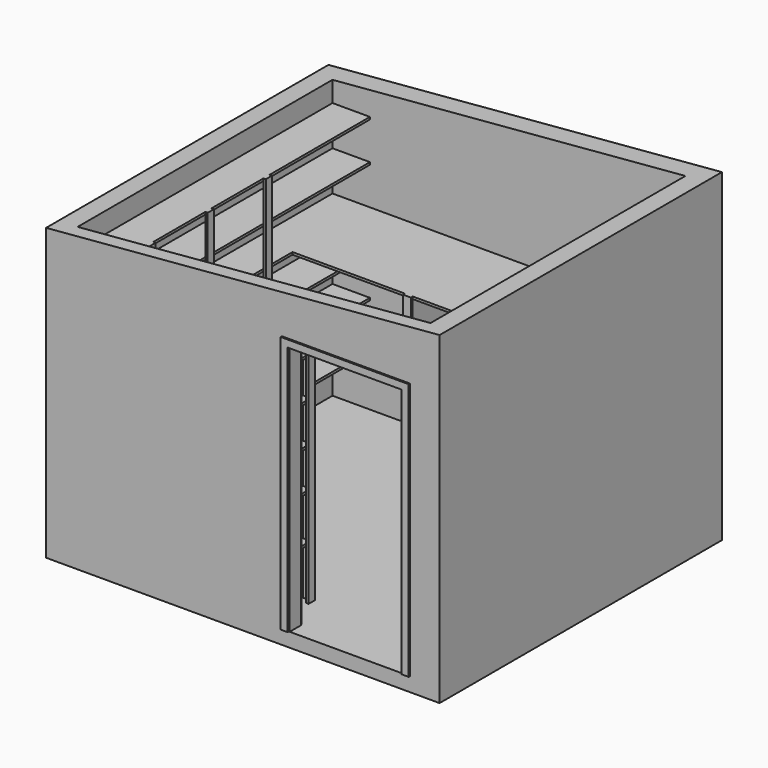
from build123d import *

# Parameters (mm, degrees)
F0_W      = 2590.8
F0_H      = 2520.95
F1_DEPTH  = 165.1
F2_W      = 3035.3
F2_H      = 2520.95
F3_DEPTH  = 114.3
F4_W      = 3035.3
F4_H      = 2520.95
F5_DEPTH  = 165.1
F6_W      = 2870.2
F6_H      = 2520.95
F7_DEPTH  = 165.1
F10_DEPTH = 2870.201
F8_W      = 914.4
F8_H      = 2032
F11_DEPTH = 114.3
F12_W     = 3200.4
F12_H     = 2870.2
F13_DEPTH = 114.3
F15_DEPTH = 12.7
F18_W     = 1651
F18_H     = 19.05
F19_DEPTH = 304.8
F20_W     = 1651
F20_H     = 38.1
F21_DEPTH = 19.05
F22_W     = 19.05
F22_H     = 63.5
F22_W_2   = 63.5
F22_H_2   = 19.05
F23_DEPTH = 2095.5
F24_W     = 2286
F24_H     = 19.05
F25_DEPTH = 304.8
F26_W     = 1422.4
F26_H     = 787.4
F26_W_2   = 990.6
F27_DEPTH = 990.6
F28_W     = 19.05
F28_H     = 787.4
F28_W_2   = 63.5
F28_H_2   = 19.05
F29_DEPTH = 1447.8
F30_W     = 19.05
F30_H     = 787.4
F31_DEPTH = 19.05
F32_W     = 2565.4
F32_H     = 787.4
F33_DEPTH = 19.05
F34_W     = 1631.95
F34_H     = 19.05
F35_DEPTH = 787.4


# Not quite as in the source:
# - a pattern or mirror of a feature is missing from the dataset's text; its kind, count and spacing are read off the source's solid


with BuildPart() as f1:
    # F0 (on Right) → F1 (new body)
    with BuildSketch(Plane.YZ):
        with Locations((1295.4, 1260.475)):
            Rectangle(F0_W, F0_H)
    extrude(amount=F1_DEPTH)

    # F2 (on face) → F3 (join)
    with BuildSketch(Plane.XZ):
        with Locations((1517.65, 1260.475)):
            Rectangle(F2_W, F2_H)
    extrude(amount=F3_DEPTH)

    # F4 (on face) → F5 (join)
    with BuildSketch(Plane(origin=(0, 2590.8, 0), x_dir=(-1, 0, 0), z_dir=(0, 1, 0))):
        with Locations((-1517.65, 1260.475)):
            Rectangle(F4_W, F4_H)
    extrude(amount=F5_DEPTH)

    # F6 (on face) → F7 (join)
    with BuildSketch(Plane.YZ.offset(3035.3)):
        with Locations((1320.8, 1260.475)):
            Rectangle(F6_W, F6_H)
    extrude(amount=F7_DEPTH)

    # F9 (on face) → F10 (cut, through all)
    with BuildSketch(Plane.XZ.offset(114.3)):
        Polygon((0, 2520.95), (0, 2247.9), (3200.4, 2520.95), align=None)
    extrude(amount=-F10_DEPTH, mode=Mode.SUBTRACT)

    # F8 (on face) → F11 (cut)
    with BuildSketch(Plane.XZ.offset(114.3)):
        with Locations((2438.4, 1016)):
            Rectangle(F8_W, F8_H)
    extrude(amount=-F11_DEPTH, mode=Mode.SUBTRACT)

    # F12 (on face) → F13 (join)
    with BuildSketch(Plane(origin=(0, 0, 0), x_dir=(1, 0, 0), z_dir=(0, 0, -1))):
        with Locations((1600.2, -1320.8)):
            Rectangle(F12_W, F12_H)
    extrude(amount=F13_DEPTH)

    # F14 (on face) → F15 (join)
    with BuildSketch(Plane(origin=(0, 0, 0), x_dir=(-1, 0, 0), z_dir=(0, 1, 0))):
        Polygon((-1974.85, 2038.35), (-1974.85, 0), (-1917.7, 0), (-1917.7, 2095.5), (-2959.1, 2095.5), (-2959.1, 0), (-2901.95, 0), (-2901.95, 2038.35), align=None)
    f15 = extrude(amount=F15_DEPTH)

    # F15_copies: F15 across plane
    add(f15.mirror(Plane(origin=(0, -57.15, 0), x_dir=(0, 0, -1), z_dir=(0, -1, 0))))

    # F18 (on face) → F19 (join)
    with BuildSketch(Plane(origin=(0, 0, 0), x_dir=(-1, 0, 0), z_dir=(0, 1, 0))):
        with Locations((-990.6, 415.925)):
            Rectangle(F18_W, F18_H)
        with Locations((-990.6, 790.575)):
            Rectangle(F18_W, F18_H)
        with Locations((-990.6, 1114.425)):
            Rectangle(F18_W, F18_H)
        with Locations((-990.6, 1438.275)):
            Rectangle(F18_W, F18_H)
        with Locations((-990.6, 1762.125)):
            Rectangle(F18_W, F18_H)
        with Locations((-990.6, 2085.975)):
            Rectangle(F18_W, F18_H)
    extrude(amount=F19_DEPTH)

    # F20 (on face) → F21 (join)
    with BuildSketch(Plane(origin=(0, 0, 0), x_dir=(-1, 0, 0), z_dir=(0, 1, 0))):
        with Locations((-990.6, 2057.4)):
            Rectangle(F20_W, F20_H)
        with Locations((-990.6, 1733.55)):
            Rectangle(F20_W, F20_H)
        with Locations((-990.6, 1409.7)):
            Rectangle(F20_W, F20_H)
        with Locations((-990.6, 1085.85)):
            Rectangle(F20_W, F20_H)
        with Locations((-990.6, 387.35)):
            Rectangle(F20_W, F20_H)
        with Locations((-990.6, 762)):
            Rectangle(F20_W, F20_H)
    extrude(amount=F21_DEPTH)

    # F22 (on face) → F23 (join)
    with BuildSketch(Plane.XY):
        with Locations((1825.625, 31.75)):
            Rectangle(F22_W, F22_H)
        Polygon((1816.1, 260.35), (1835.15, 260.35), (1835.15, 323.85), (1816.1, 323.85), (1816.1, 304.8), align=None)
        with Locations((1784.35, 314.325)):
            Rectangle(F22_W_2, F22_H_2)
        with Locations((1358.9, 314.325)):
            Rectangle(F22_W_2, F22_H_2)
        Polygon((533.4, 304.8), (533.4, 323.85), (488.95, 323.85), (469.9, 323.85), (469.9, 304.8), align=None)
        with Locations((479.425, 355.6)):
            Rectangle(F22_W, F22_H)
        with Locations((479.425, 949.325)):
            Rectangle(F22_W, F22_H)
        with Locations((479.425, 1539.875)):
            Rectangle(F22_W, F22_H)
        with Locations((927.1, 314.325)):
            Rectangle(F22_W_2, F22_H_2)
    extrude(amount=F23_DEPTH)

    # F24 (on face) → F25 (join)
    with BuildSketch(Plane.YZ.offset(165.1)):
        with Locations((1447.8, 2085.975)):
            Rectangle(F24_W, F24_H)
        with Locations((1447.8, 1762.125)):
            Rectangle(F24_W, F24_H)
        with Locations((1447.8, 1438.275)):
            Rectangle(F24_W, F24_H)
        with Locations((1447.8, 415.925)):
            Rectangle(F24_W, F24_H)
        with Locations((1447.8, 790.575)):
            Rectangle(F24_W, F24_H)
        with Locations((1447.8, 1114.425)):
            Rectangle(F24_W, F24_H)
    extrude(amount=F25_DEPTH)

    # F26 (on face) → F27 (cut)
    with BuildSketch(Plane.XY.offset(425.45)):
        with Locations((1333.5, 2197.1)):
            Rectangle(F26_W, F26_H)
        with Locations((2540, 2197.1)):
            Rectangle(F26_W_2, F26_H)
    extrude(amount=F27_DEPTH, mode=Mode.SUBTRACT)

    # F28 (on face) → F29 (join)
    with BuildSketch(Plane.XY):
        Polygon((1447.8, 1803.4), (1403.35, 1803.4), (1384.3, 1803.4), (1384.3, 1784.35), (1447.8, 1784.35), align=None)
        with Locations((1393.825, 2197.1)):
            Rectangle(F28_W, F28_H)
        with Locations((3003.55, 1793.875)):
            Rectangle(F28_W_2, F28_H_2)
    extrude(amount=F29_DEPTH)

    # F30 (on face) → F31 (cut)
    with BuildSketch(Plane.XY.offset(1447.8)):
        with Locations((1393.825, 2197.1)):
            Rectangle(F30_W, F30_H)
    extrude(amount=-F31_DEPTH, mode=Mode.SUBTRACT)

    # F32 (on face) → F33 (join)
    with BuildSketch(Plane.XY.offset(1428.75)):
        with Locations((1752.6, 2197.1)):
            Rectangle(F32_W, F32_H)
    extrude(amount=F33_DEPTH)

    # F34 (on face) → F35 (join)
    with BuildSketch(Plane.XZ.offset(-2590.8)):
        with Locations((2219.325, 415.925)):
            Rectangle(F34_W, F34_H)
    extrude(amount=F35_DEPTH)


solid = f1.part
